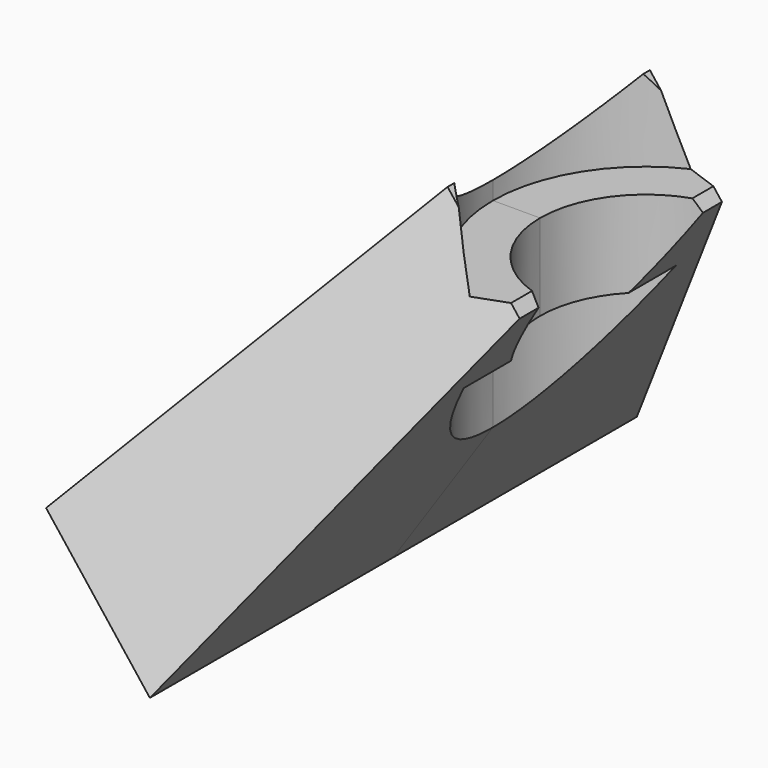
from build123d import *

# Parameters (mm, degrees)
F7_W = 22.86
F7_H = 12.7
F9_W = 9.4991559163
F9_H = 8.810961619


# Not quite as in the source:
# - a feature names something its author has since deleted; it is built from what else it names
# - the program builds the solid bodies; features that only make, move or delete a surface that nothing else refers to are left out


with BuildPart() as f10:
    # F7 (on line) → F10 section 0
    with BuildSketch(Plane(origin=(-22.86, 0, -17.78), x_dir=(0, -1, 0), z_dir=(-0.7893522174, 0, -0.6139406135))):
        with Locations((11.43, 0)):
            Rectangle(F7_W, F7_H)
    # F9 (on line) → F10 section 1
    with BuildSketch(Plane(origin=(0, 0, 0), x_dir=(0, -1, 0), z_dir=(-0.7893522174, 0, -0.6139406135))):
        with Locations((4.7495779581, 7.4622994289)):
            Rectangle(F9_W, F9_H)
    loft()

    # F11 (on Front) → F12 (revolve, cut)
    with BuildSketch(Plane.XZ):
        Polygon((-11.4808, 13.2924560457), (-11.4808, 4.7625), (-11.4808, 3.2385), (-7.9375, 3.2385), (-7.9375, -3.2385), (-11.4808, -3.2385), (-11.4808, -4.7625), (-11.4808, -25.4), (0, -25.4), (0, 0), (0, 13.2924560457), align=None)
    revolve(axis=Axis((0, 0, -12.7), (0, 0, 1)), mode=Mode.SUBTRACT)


with BuildPart() as f13_1:
    # F13: instance of F10
    add(f10.part.mirror(Plane.XZ))


solid = Compound([f10.part, f13_1.part])
